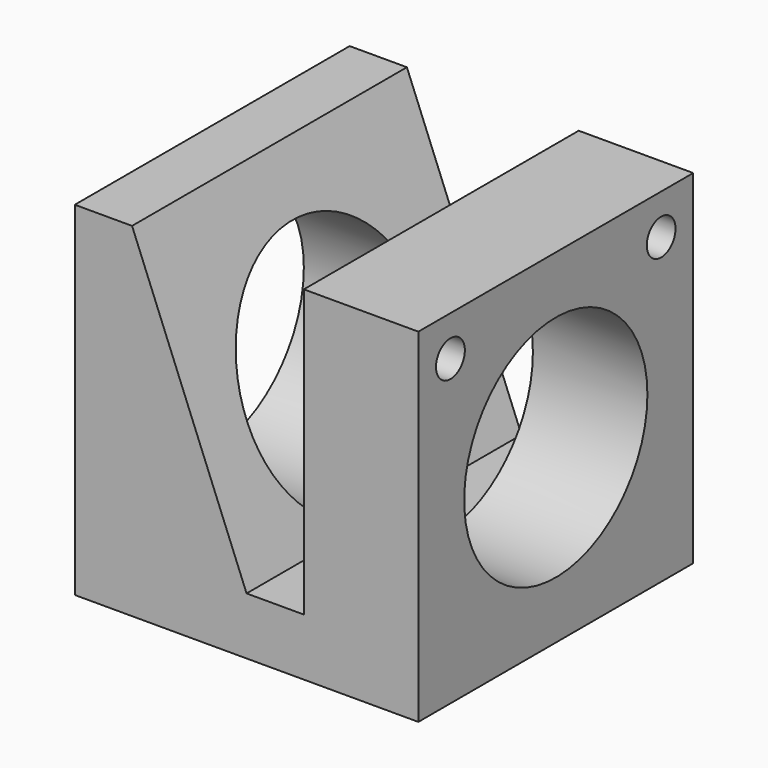
from build123d import *

# Parameters (mm, degrees)
F1_DEPTH = 19.05
F2_R     = 12.7
F3_DEPTH = 38.1
F2_R_2   = 1.9939
F2_R_3   = 1.99898
F4_DEPTH = 12.7


# Not quite as in the source:
# - a feature names something its author has since deleted; it is built from what else it names


with BuildPart() as f1:
    # F0 (on Front) → F1 (new body, symmetric)
    with BuildSketch(Plane.XZ):
        Polygon((19.05, -19.05), (19.05, 19.05), (6.35, 19.05), (6.35, -12.7), (0, -12.7), (-12.7, 19.05), (-19.05, 19.05), (-19.05, -19.05), align=None)
    extrude(amount=F1_DEPTH, both=True)

    # F2 (on face) → F3 (cut)
    with BuildSketch(Plane.YZ.offset(19.05)):
        Circle(F2_R)
    extrude(amount=-F3_DEPTH, mode=Mode.SUBTRACT)

    # F2 (on face) → F4 (cut)
    with BuildSketch(Plane.YZ.offset(19.05)):
        with Locations((14.605, 14.605)):
            Circle(F2_R_2)
        with Locations((-14.605, 14.605)):
            Circle(F2_R_3)
    extrude(amount=-F4_DEPTH, mode=Mode.SUBTRACT)


solid = f1.part
